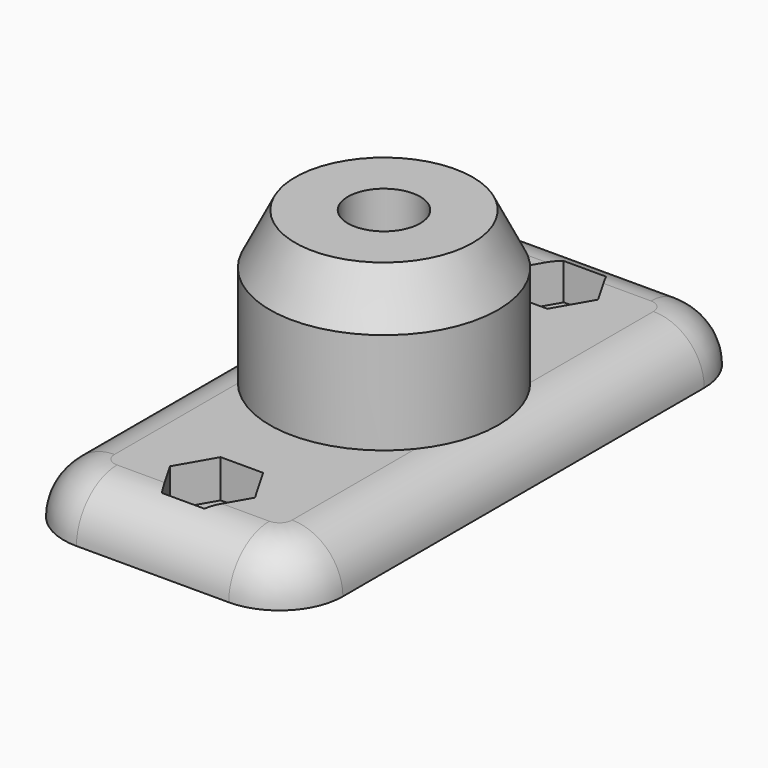
from build123d import *

# Parameters (mm, degrees)
F2_W      = 22
F2_H      = 45.6
F2_R      = 1.7
F3_DEPTH  = 4
F4_R      = 5
F5_R      = 3.99999
F6_DEPTH  = 3
F8_R      = 9
F9_DEPTH  = 12
F10_R     = 2.85
F11_DEPTH = 8
F12_R     = 2.15
F13_DEPTH = 8
F13_TAPER = -0.5
F14_SIZE2 = 4
F14_SIZE  = 2


# Not quite as in the source:
# - a fillet or chamfer is up to 0.001 mm smaller than in the source, because OpenCascade refuses the exact size
# - a feature names something its author has since deleted; it is built from what else it names


with BuildPart() as f3:
    # F2 (on Top) → F3 (new body)
    with BuildSketch(Plane.XY):
        Rectangle(F2_W, F2_H)
        Polygon((3.3486315613, -16.9), (1.6743157806, -19.8), (-1.6743157806, -19.8), (-3.3486315613, -16.9), (-1.6743157806, -14), (1.6743157806, -14), align=None, mode=Mode.SUBTRACT)
        Circle(F2_R, mode=Mode.SUBTRACT)
        Polygon((1.6743157806, 19.8), (3.3486315613, 16.9), (1.6743157806, 14), (-1.6743157806, 14), (-3.3486315613, 16.9), (-1.6743157806, 19.8), align=None, mode=Mode.SUBTRACT)
        Polygon((1.6743157806, 14), (3.3486315613, 16.9), (1.6743157806, 19.8), (-1.6743157806, 19.8), (-3.3486315613, 16.9), (-1.6743157806, 14), align=None)
        with Locations((0, 16.9)):
            Circle(F2_R, mode=Mode.SUBTRACT)
        Circle(F2_R)
        Polygon((-1.6743157806, -19.8), (1.6743157806, -19.8), (3.3486315613, -16.9), (1.6743157806, -14), (-1.6743157806, -14), (-3.3486315613, -16.9), align=None)
        with Locations((0, -16.9)):
            Circle(F2_R, mode=Mode.SUBTRACT)
    extrude(amount=-F3_DEPTH)

    # F4
    f4_edges = [f3.edges().sort_by_distance(p)[0] for p in [
        (-11, 22.8, -2),
        (11, 22.8, -2),
        (11, -22.8, -2),
        (-11, -22.8, -2),
    ]]
    fillet(f4_edges, radius=F4_R)

    # F5 (radius 4 in the source; OpenCascade refuses exactly that, so slightly less here)
    f5_edges = [f3.edges().sort_by_distance(p)[0] for p in [
        (-11, 0, 0),
        (0, -22.8, 0),
        (-9.535534, -21.335534, 0),
        (9.535534, -21.335534, 0),
        (11, 0, 0),
        (9.535534, 21.335534, 0),
        (0, 22.8, 0),
        (-9.535534, 21.335534, 0),
    ]]
    fillet(f5_edges, radius=F5_R)

    # F2 (on Top) → F6 (cut)
    with BuildSketch(Plane.XY):
        Polygon((1.6743157806, 14), (3.3486315613, 16.9), (1.6743157806, 19.8), (-1.6743157806, 19.8), (-3.3486315613, 16.9), (-1.6743157806, 14), align=None)
        with Locations((0, 16.9)):
            Circle(F2_R, mode=Mode.SUBTRACT)
        Polygon((-1.6743157806, -19.8), (1.6743157806, -19.8), (3.3486315613, -16.9), (1.6743157806, -14), (-1.6743157806, -14), (-3.3486315613, -16.9), align=None)
        with Locations((0, -16.9)):
            Circle(F2_R, mode=Mode.SUBTRACT)
    extrude(amount=-F6_DEPTH, mode=Mode.SUBTRACT)

    # F8 (on line) → F9 (join)
    with BuildSketch(Plane.XY):
        Circle(F8_R)
    extrude(amount=F9_DEPTH)

    # F10 (on face) → F11 (cut)
    with BuildSketch(Plane.XY.offset(12)):
        Circle(F10_R)
    extrude(amount=-F11_DEPTH, mode=Mode.SUBTRACT)

    # F12 (on face) → F13 (cut, through all)
    with BuildSketch(Plane.XY.offset(4)):
        Circle(F12_R)
    extrude(amount=-F13_DEPTH, taper=F13_TAPER, mode=Mode.SUBTRACT)

    # F14
    f14_edges = [f3.edges().sort_by_distance(p)[0] for p in [
        (-9, 0, 12),
    ]]
    f14_side = f3.faces().sort_by_distance((-8.745442, 0, 12))[0]
    chamfer(f14_edges, length=F14_SIZE, length2=F14_SIZE2, reference=f14_side)


solid = f3.part
